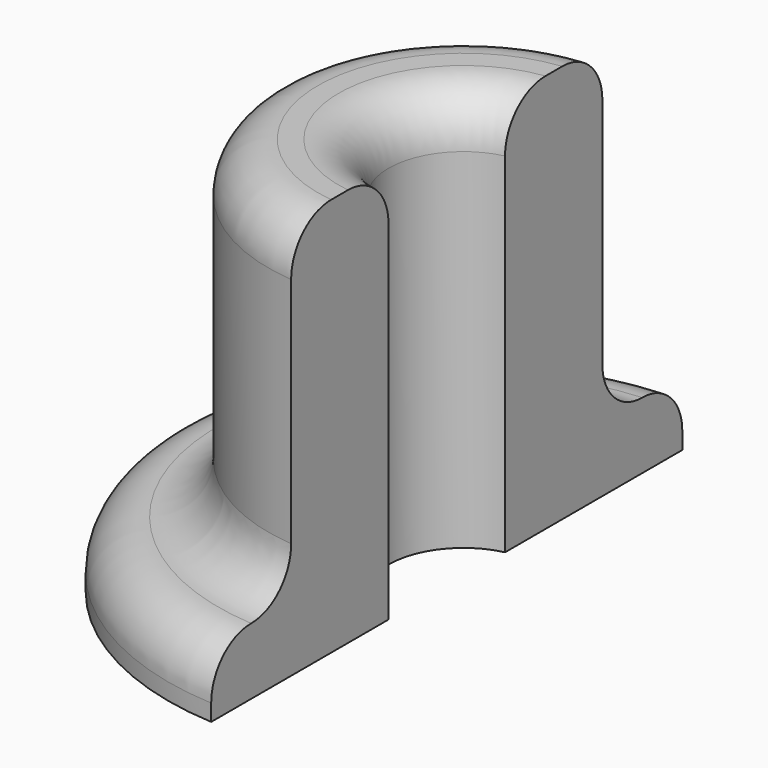
from build123d import *

# Parameters (mm, degrees)
F1_DEPTH = 12
F2_DEPTH = 2
F3_R     = 1.49999


# Not quite as in the source:
# - a fillet or chamfer is up to 0.001 mm smaller than in the source, because OpenCascade refuses the exact size


with BuildPart() as f1:
    # F0 (on Top) → F1 (new body)
    with BuildSketch(Plane.XY):
        with BuildLine():
            ThreePointArc((-0.5, -2.1937410968), (-2.25, 0), (-0.5, 2.1937410968))
            Line((-0.5, 2.1937410968), (-0.5, 5.853684737))
            ThreePointArc((-0.5, 5.853684737), (-5.875, 0), (-0.5, -5.853684737))
            Line((-0.5, -5.853684737), (-0.5, -2.1937410968))
        make_face()
    extrude(amount=F1_DEPTH)

    # F0 (on Top) → F2 (join)
    with BuildSketch(Plane.XY):
        with BuildLine():
            ThreePointArc((-0.5, -5.853684737), (-5.875, 0), (-0.5, 5.853684737))
            Line((-0.5, 5.853684737), (-0.5, 8.8609042992))
            ThreePointArc((-0.5, 8.8609042992), (-8.875, 0), (-0.5, -8.8609042992))
            Line((-0.5, -8.8609042992), (-0.5, -5.853684737))
        make_face()
    extrude(amount=F2_DEPTH)

    # F3 (radius 1.5 in the source; OpenCascade refuses exactly that, so slightly less here)
    f3_edges = [f1.edges().sort_by_distance(p)[0] for p in [
        (-5.875, 0, 2),
        (-8.875, 0, 2),
        (-5.875, 0, 12),
        (-2.25, 0, 12),
    ]]
    fillet(f3_edges, radius=F3_R)


solid = f1.part
